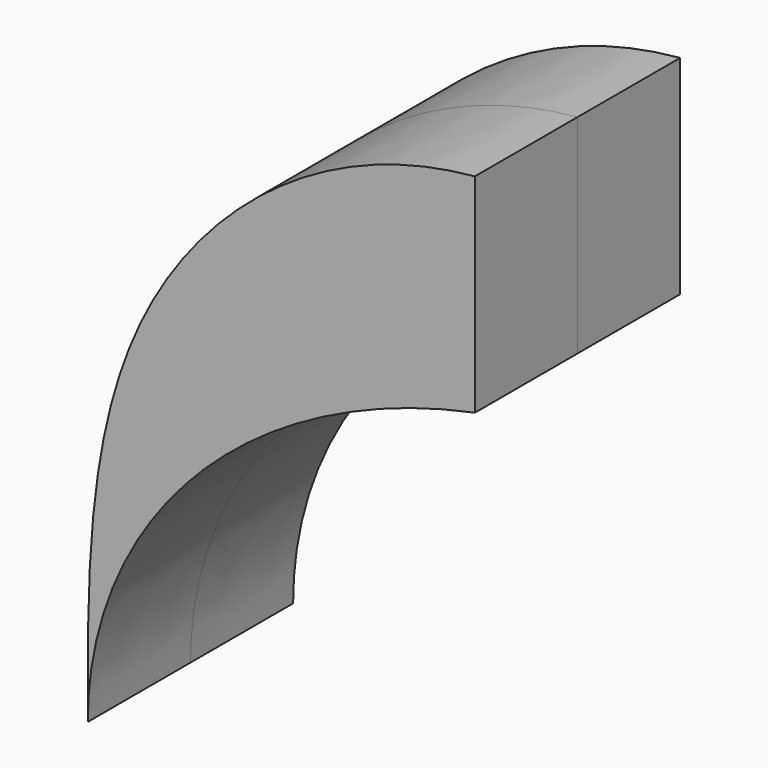
from build123d import *

# Parameters (mm, degrees)
F1_DEPTH = 12.5


with BuildPart() as f1:
    # F0 (on Front) → F1 (new body, symmetric)
    with BuildSketch(Plane.XZ):
        with BuildLine():
            add(Edge.make_bspline(
                [(-50, 0), (-50.0407398567, 12.683133187), (-50.1235942028, 38.4773502806), (-27.2922330655, 57.7014225305), (-12.3019693419, 59.0356364846)],
                knots=[0, 0, 0, 0, 0.2331907275, 0.4742497111, 0.4742497111, 0.4742497111, 0.4742497111], degree=3))
            add(Edge.make_bspline(
                [(-12.2957733851, 38.7716511435), (-50, 31.1190061835), (-50, 0)],
                knots=[1.8192603775, 1.8192603775, 1.8192603775, 3.1415926536, 3.1415926536, 3.1415926536], degree=2, weights=[1, 0.7892767156, 1]))
            add(Edge.make_bspline(
                [(-12.3019693419, 59.0356364846), (-12.2990112342, 52.4271155186), (-12.2963394707, 45.8169153956), (-12.2957733851, 38.7716511435)],
                knots=[0, 0, 0, 0, 0.2005574694, 0.2005574694, 0.2005574694, 0.2005574694], degree=3))
        make_face()
    extrude(amount=F1_DEPTH, both=True)


solid = f1.part
